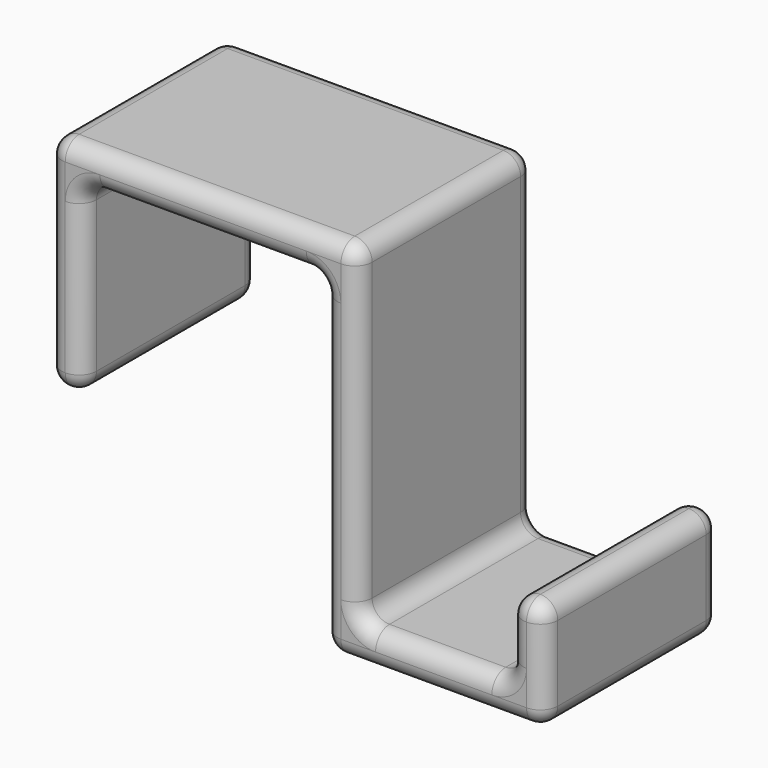
from build123d import *

# Parameters (mm, degrees)
F1_DEPTH = 50.8
F2_R     = 3.99999


# Not quite as in the source:
# - a fillet or chamfer is up to 0.001 mm smaller than in the source, because OpenCascade refuses the exact size


with BuildPart() as f1:
    # F0 (on Front) → F1 (new body)
    with BuildSketch(Plane.XZ):
        Polygon((71.5625, 0), (0, 0), (0, -50.8), (8, -50.8), (8, -8), (63.5625, -8), (63.5625, -84.2), (114.3625, -84.2), (114.3625, -58.8), (106.3625, -58.8), (106.3625, -76.2), (71.5625, -76.2), align=None)
    extrude(amount=F1_DEPTH)

    # F2 (radius 4 in the source; OpenCascade refuses exactly that, so slightly less here)
    f2_edges = [f1.edges().sort_by_distance(p)[0] for p in [
        (0, -25.4, 0),
        (71.5625, -25.4, 0),
        (71.5625, -25.4, -76.2),
        (106.3625, -25.4, -76.2),
        (71.5625, -50.8, -38.1),
        (71.5625, 0, -38.1),
        (110.3625, 0, -58.8),
        (114.3625, -25.4, -58.8),
        (110.3625, -50.8, -58.8),
        (106.3625, -25.4, -58.8),
        (114.3625, -25.4, -84.2),
        (114.3625, -50.8, -71.5),
        (114.3625, 0, -71.5),
        (88.9625, 0, -84.2),
        (88.9625, -50.8, -84.2),
        (63.5625, -25.4, -84.2),
        (63.5625, -50.8, -46.1),
        (63.5625, 0, -46.1),
        (0, 0, -25.4),
        (0, -50.8, -25.4),
        (0, -25.4, -50.8),
        (88.9625, 0, -76.2),
        (8, 0, -29.4),
        (8, -50.8, -29.4),
        (35.78125, -50.8, -8),
        (88.9625, -50.8, -76.2),
        (106.3625, 0, -67.5),
        (4, -50.8, -50.8),
        (106.3625, -50.8, -67.5),
        (8, -25.4, -50.8),
        (35.78125, -50.8, 0),
        (35.78125, 0, 0),
        (8, -25.4, -8),
        (63.5625, -25.4, -8),
        (4, 0, -50.8),
        (35.78125, 0, -8),
    ]]
    fillet(f2_edges, radius=F2_R)


solid = f1.part
